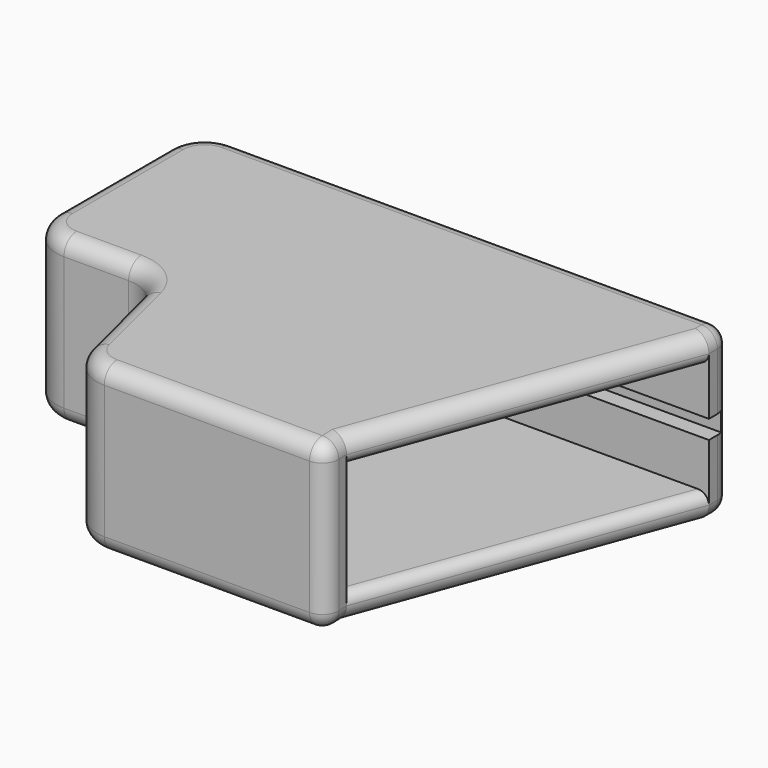
from build123d import *

# Parameters (mm, degrees)
F1_DEPTH = 21
F4_DEPTH = 5
F5_DEPTH = 5
F6_R     = 7
F7_R     = 3
F9_DEPTH = 3
F10_R    = 1.99999


# Not quite as in the source:
# - a fillet or chamfer is up to 0.001 mm smaller than in the source, because OpenCascade refuses the exact size


with BuildPart() as f1:
    # F0 (on Top) → F1 (new body)
    with BuildSketch(Plane.XY):
        Polygon((-23.5, 30), (71.5, 30), (71.5, 35), (-28.5, 35), (-28.5, -5), (-3.906596233, -5), (3.1079638678, -33.1388689644), (50.2020280941, -33.1388689644), (50.0145601007, -28.1388689644), (7.0145601007, -28.1388689644), (0, 0), (-23.5, 0), align=None)
    extrude(amount=F1_DEPTH)

    # F3 (on face) → F4 (join)
    with BuildSketch(Plane.XY.offset(21)):
        Polygon((71.5, 35), (-28.5, 35), (-28.5, -5), (-3.906596233, -5), (3.1079638678, -33.1388689644), (50.2020280941, -33.1388689644), (50.0145601007, -28.1388689644), (71.5, 30), align=None)
    extrude(amount=F4_DEPTH)

    # F2 (on face) → F5 (join)
    with BuildSketch(Plane(origin=(0, 0, 0), x_dir=(1, 0, 0), z_dir=(0, 0, -1))):
        Polygon((-28.5, -35), (71.5, -35), (71.5, -30), (50.0145601007, 28.1388689644), (50.2020280941, 33.1388689644), (3.1079638678, 33.1388689644), (-3.906596233, 5), (-28.5, 5), align=None)
    extrude(amount=F5_DEPTH)

    # F6
    f6_edges = [f1.edges().sort_by_distance(p)[0] for p in [
        (0, 0, 10.5),
        (-3.906596, -5, 10.5),
        (7.01456, -28.138869, 10.5),
        (3.107964, -33.138869, 10.5),
        (-28.5, -5, 10.5),
        (-28.5, 35, 10.5),
        (-23.5, 0, 10.5),
    ]]
    fillet(f6_edges, radius=F6_R)

    # F7
    f7_edges = [f1.edges().sort_by_distance(p)[0] for p in [
        (25, 35, 26),
        (25, 35, -5),
        (71.5, 35, 10.5),
        (-26.449747, 32.949747, 26),
        (71.5, 32.5, 26),
        (-28.5, 15, 26),
        (60.75728, 0.930566, 26),
        (-26.449747, -2.949747, 26),
        (50.108294, -30.638869, 26),
        (-15.437915, -5, 26),
        (29.389613, -33.138869, 26),
        (-5.066085, -6.484015, 26),
        (4.267453, -31.654854, 26),
        (-0.399316, -19.069434, 26),
        (-15.437915, -5, -5),
        (-5.066085, -6.484015, -5),
        (-26.449747, -2.949747, -5),
        (-0.399316, -19.069434, -5),
        (-28.5, 15, -5),
        (4.267453, -31.654854, -5),
        (-26.449747, 32.949747, -5),
        (29.389613, -33.138869, -5),
        (50.108294, -30.638869, -5),
        (71.5, 32.5, -5),
        (60.75728, 0.930566, -5),
        (50.202028, -33.138869, 10.5),
    ]]
    fillet(f7_edges, radius=F7_R)

    # F8 (on face) → F9 (cut)
    with BuildSketch(Plane.XZ.offset(-30)):
        Polygon((-23.5, 12.25), (-23.5, 10.5), (-23.5, 8.75), (74.1642639041, 8.75), (74.1642639041, 12.25), align=None)
    extrude(amount=-F9_DEPTH, mode=Mode.SUBTRACT)

    # F10 (radius 2 in the source; OpenCascade refuses exactly that, so slightly less here)
    f10_edges = [f1.edges().sort_by_distance(p)[0] for p in [
        (60.75728, 0.930566, 21),
        (60.75728, 0.930566, 0),
    ]]
    fillet(f10_edges, radius=F10_R)


solid = f1.part
